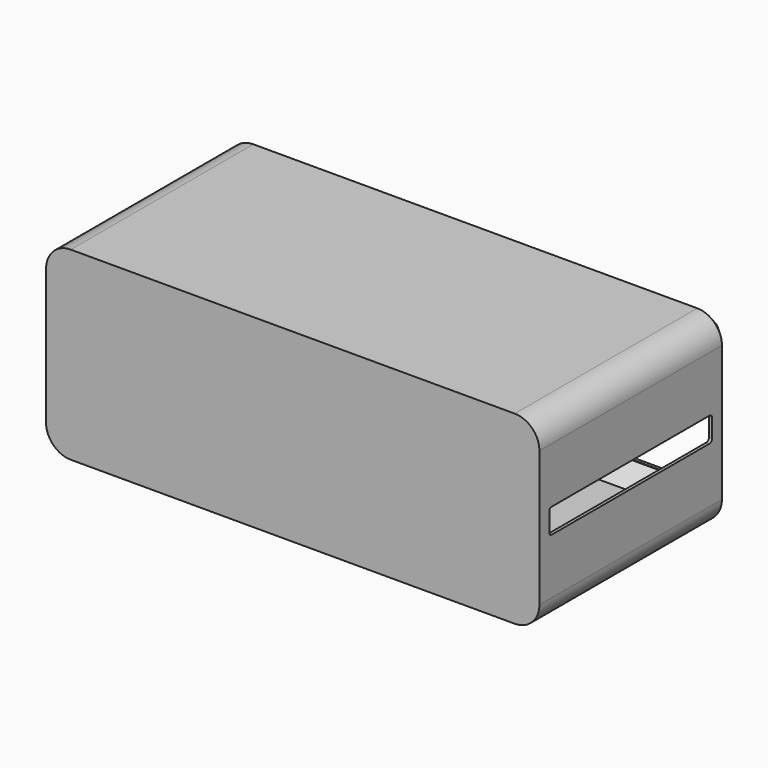
from build123d import *

# Parameters (mm, degrees)
F0_W     = 800
F0_H     = 300
F1_DEPTH = 400
F2_R     = 40
F3_SIZE  = 30
F5_DEPTH = 5
F6_T     = 5
F8_DEPTH = 800.001


# Not quite as in the source:
# - a shell that OpenCascade refuses in one call is made with other operations: the cavity is built on its own and cut out


with BuildPart() as f1:
    # F0 (on Front) → F1 (new body)
    with BuildSketch(Plane.XZ):
        Rectangle(F0_W, F0_H)
    extrude(amount=F1_DEPTH)

    # F2
    f2_edges = [f1.edges().sort_by_distance(p)[0] for p in [
        (400, -200, 150),
        (-400, -200, 150),
        (400, -200, -150),
        (-400, -200, -150),
    ]]
    fillet(f2_edges, radius=F2_R)

    # F3
    f3_edges = [f1.edges().sort_by_distance(p)[0] for p in [
        (0, 0, 150),
        (0, 0, -150),
        (-388.284271, 0, -138.284271),
        (388.284271, 0, -138.284271),
        (-400, 0, 0),
        (400, 0, 0),
        (-388.284271, 0, 138.284271),
        (388.284271, 0, 138.284271),
    ]]
    chamfer(f3_edges, length=F3_SIZE)

    # F4 (on face) → F5 (cut)
    with BuildSketch(Plane(origin=(0, 0, 0), x_dir=(-1, 0, 0), z_dir=(0, 1, 0))):
        with BuildLine():
            Line((366.9999986887, -110), (366.9999986887, 110))
            ThreePointArc((366.9999986887, 110), (364.9497465411, 114.9497465411), (360, 116.9999986887))
            Line((360, 116.9999986887), (-360, 116.9999986887))
            ThreePointArc((-360, 116.9999986887), (-364.9497465411, 114.9497465411), (-366.9999986887, 110))
            Line((-366.9999986887, 110), (-366.9999986887, -110))
            ThreePointArc((-366.9999986887, -110), (-364.9497465411, -114.9497465411), (-360, -116.9999986887))
            Line((-360, -116.9999986887), (360, -116.9999986887))
            ThreePointArc((360, -116.9999986887), (364.9497465411, -114.9497465411), (366.9999986887, -110))
        make_face()
    extrude(amount=-F5_DEPTH, mode=Mode.SUBTRACT)

    # F6: shell of thickness 5, made by hand


with BuildPart() as f6_core1:
    # F6_t2: copy of F1
    add(f1.part)

    # the walls: a layer under each face that stays
    f6_faces = [f6_core1.faces().sort_by_distance(p)[0] for p in [
        (0, -215, -150),
        (-388.2842712475, -215, -138.2842712475),
        (0, -15, -135),
        (0, -400, 0),
        (388.2842712475, -215, -138.2842712475),
        (-377.6776695297, -15, -127.6776695297),
        (-400, -215, 0),
        (254.375, 0, -117.037037037),
        (377.6776695297, -15, -127.6776695297),
        (400, -215, 0),
        (-388.2842712475, -215, 138.2842712475),
        (388.2842712475, -215, 138.2842712475),
        (0, -215, 150),
        (-385, -15, 0),
        (0, -15, 135),
        (377.6776695297, -15, 127.6776695297),
        (-377.6776695297, -15, 127.6776695297),
        (385, -15, 0),
        (364.9497465411, -2.5, -114.9497465411),
        (366.9999986887, -2.5, 0),
        (364.9497465411, -2.5, 114.9497465411),
        (0, -2.5, 116.9999986887),
        (-364.9497465411, -2.5, 114.9497465411),
        (-366.9999986887, -2.5, 0),
        (-364.9497465411, -2.5, -114.9497465411),
        (0, -2.5, -116.9999986887),
    ]]
    thicken(f6_faces, amount=-F6_T, mode=Mode.SUBTRACT)


with BuildPart() as f1_1:
    add(f1.part)

    # what is left inside the walls is the cavity
    f6_cavity = [f6_core1.part.solids().sort_by_distance(p)[0] for p in [
        (0, -274.023689, -144.95),
    ]]
    add(f6_cavity, mode=Mode.SUBTRACT)

    # F7 (on face) → F8 (cut, through all)
    with BuildSketch(Plane.YZ.offset(400)):
        with BuildLine():
            Line((-375, -20), (-55, -20))
            ThreePointArc((-55, -20), (-51.4644660941, -18.5355339059), (-50, -15))
            Line((-50, -15), (-50, 15))
            ThreePointArc((-50, 15), (-51.4644660941, 18.5355339059), (-55, 20))
            Line((-55, 20), (-375, 20))
            ThreePointArc((-375, 20), (-378.5355339059, 18.5355339059), (-380, 15))
            Line((-380, 15), (-380, -15))
            ThreePointArc((-380, -15), (-378.5355339059, -18.5355339059), (-375, -20))
        make_face()
    extrude(amount=-F8_DEPTH, mode=Mode.SUBTRACT)


solid = f1_1.part
